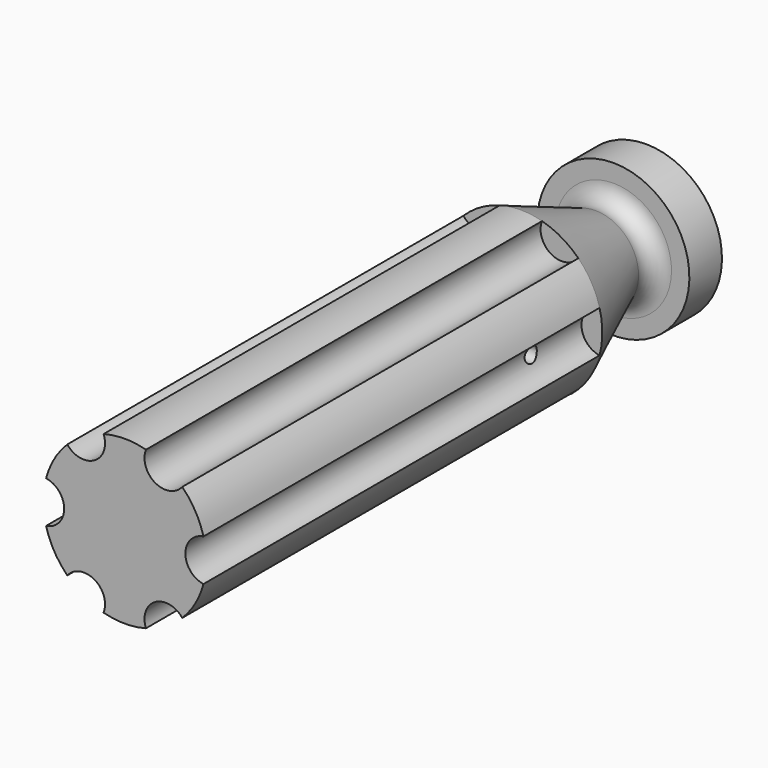
from build123d import *

# Parameters (mm, degrees)
F2_R          = 3.302
F3_DEPTH      = 77.216
F5_START      = -40.64
F4_R          = 3.175
F5_DEPTH      = 60.961
F6_R          = 1.1938
F7_DEPTH      = 25.4
F7_DEPTH_BACK = 25.4


# Not quite as in the source:
# - a feature names something its author has since deleted; it is built from what else it names


with BuildPart() as f1:
    # F0 (on Right) → F1 (revolve)
    with BuildSketch(Plane.YZ):
        with BuildLine():
            Line((0, 12.7), (0, 0))
            Line((0, 0), (101.6, 0))
            Line((101.6, 0), (101.6, 11.8551712597))
            Line((101.6, 11.8551712597), (95.25, 11.8551712597))
            Line((95.25, 11.8551712597), (95.25, 9.0634808418))
            ThreePointArc((95.25, 9.0634808418), (94.1293552402, 6.9632371008), (91.7608131807, 6.7247481879))
            Line((91.7608131807, 6.7247481879), (77.216, 12.7))
            Line((77.216, 12.7), (0, 12.7))
        make_face()
    revolve(axis=Axis((0, 50.8, 0), (0, 1, 0)))

    # F2 (on Front) → F3 (cut)
    with BuildSketch(Plane.XZ):
        with Locations((12.7568459138, 0)):
            Circle(F2_R)
        with Locations((6.3784229569, 11.0477526335)):
            Circle(F2_R)
        with Locations((-6.3784229569, 11.0477526335)):
            Circle(F2_R)
        with Locations((-12.7568459138, 0)):
            Circle(F2_R)
        with Locations((-6.3784229569, -11.0477526335)):
            Circle(F2_R)
        with Locations((6.3784229569, -11.0477526335)):
            Circle(F2_R)
    extrude(amount=-F3_DEPTH, mode=Mode.SUBTRACT)

    # F4 (on Front) → F5 (cut)
    with BuildSketch(Plane.XZ.offset(F5_START)):
        Circle(F4_R)
    extrude(amount=-F5_DEPTH, mode=Mode.SUBTRACT)

    # F6 (on Right) → F7 (cut, two sides)
    with BuildSketch(Plane.YZ) as f7_sk:
        with Locations((67.31, 0)):
            Circle(F6_R)
    extrude(amount=-F7_DEPTH, mode=Mode.SUBTRACT)
    extrude(f7_sk.sketch, amount=F7_DEPTH_BACK, mode=Mode.SUBTRACT)


solid = f1.part
